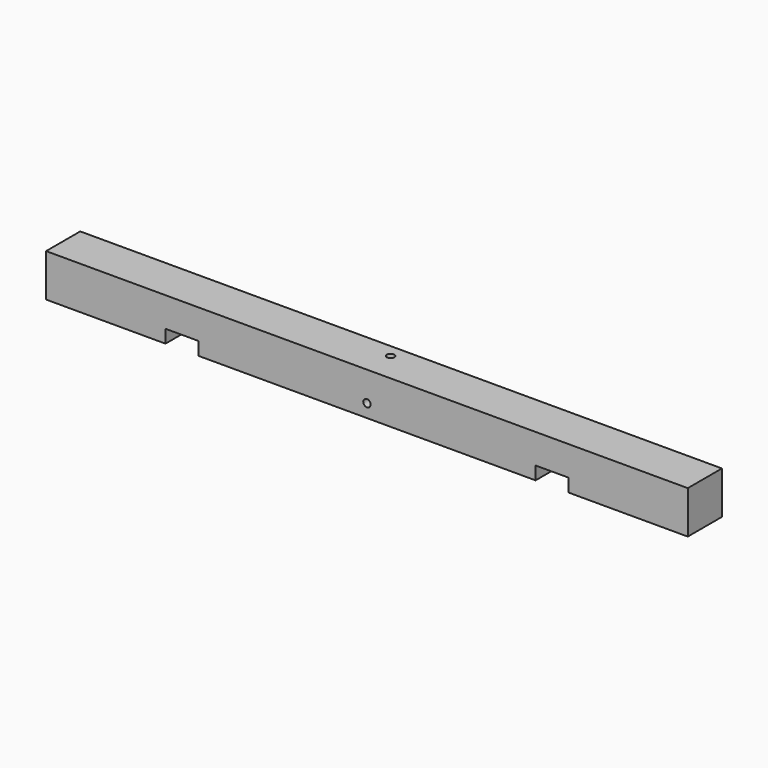
from build123d import *

# Parameters (mm, degrees)
F0_W     = 26
F0_H     = 26
F1_DEPTH = 195.5
F4_D     = 4.5
F6_D     = 4.5
F7_W     = 20
F7_H     = 8
F8_DEPTH = 26


# Not quite as in the source:
# - a pattern or mirror of a feature is missing from the dataset's text; its kind, count and spacing are read off the source's solid


with BuildPart() as f1:
    # F0 (on Right) → F1 (new body, symmetric)
    with BuildSketch(Plane.YZ):
        with Locations((0, 13)):
            Rectangle(F0_W, F0_H)
    extrude(amount=F1_DEPTH, both=True)

    # F4 (through all)
    with Locations(Plane.XZ.offset(13)):
        with Locations((0, 8)):
            Hole(F4_D / 2)

    # F6 (through all)
    with Locations(Plane(origin=(0, 0, 0), x_dir=(1, 0, 0), z_dir=(0, 0, -1))):
        with Locations((0, -5)):
            Hole(F6_D / 2)

    # F7 (on face) → F8 (cut, through all)
    with BuildSketch(Plane.XZ.offset(13)):
        with Locations((-112.75, 4)):
            Rectangle(F7_W, F7_H)
    f8 = extrude(amount=-F8_DEPTH, mode=Mode.SUBTRACT)

    # F8_copies: F8 across plane
    add(f8.mirror(Plane(origin=(0, 0, 0), x_dir=(0, 0, 1), z_dir=(1, 0, 0))), mode=Mode.SUBTRACT)


solid = f1.part
